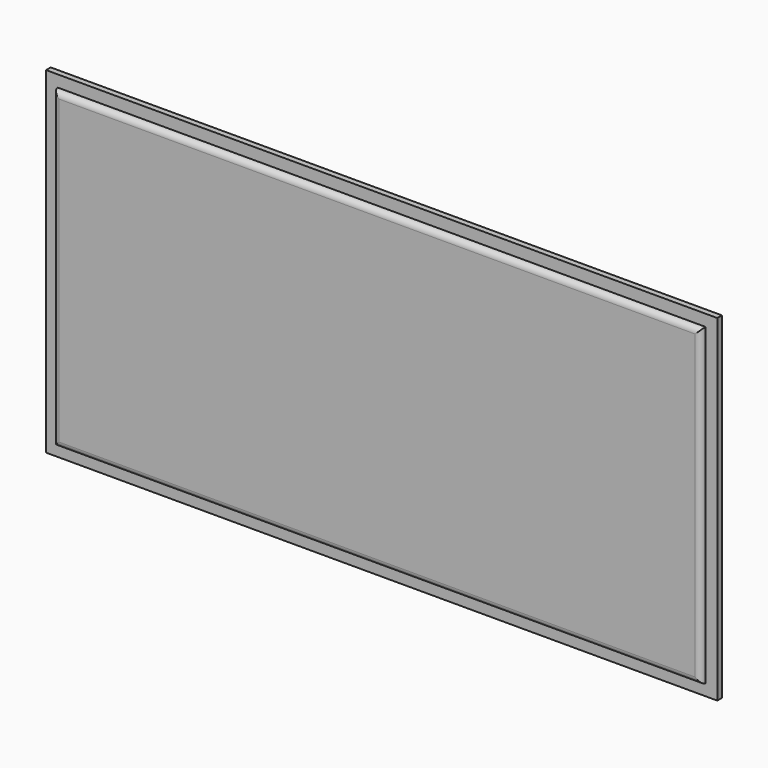
from build123d import *

# Parameters (mm, degrees)
F0_W     = 115.58
F0_H     = 58
F1_DEPTH = 1
F2_W     = 111.58
F2_H     = 54
F3_DEPTH = 1
F4_R     = 0.99999


# Not quite as in the source:
# - a fillet or chamfer is up to 0.001 mm smaller than in the source, because OpenCascade refuses the exact size
# - a feature names something its author has since deleted; it is built from what else it names


with BuildPart() as f1:
    # F0 (on Front) → F1 (new body)
    with BuildSketch(Plane.XZ):
        with Locations((57.79, 29)):
            Rectangle(F0_W, F0_H)
    extrude(amount=F1_DEPTH)

    # F2 (on face) → F3 (join)
    with BuildSketch(Plane.XZ.offset(1)):
        with Locations((57.79, 29)):
            Rectangle(F2_W, F2_H)
    extrude(amount=F3_DEPTH)

    # F4 (radius 1 in the source; OpenCascade refuses exactly that, so slightly less here)
    f4_edges = [f1.edges().sort_by_distance(p)[0] for p in [
        (57.79, -2, 56),
        (2, -2, 29),
        (57.79, -2, 2),
        (113.58, -2, 29),
    ]]
    fillet(f4_edges, radius=F4_R)


solid = f1.part
